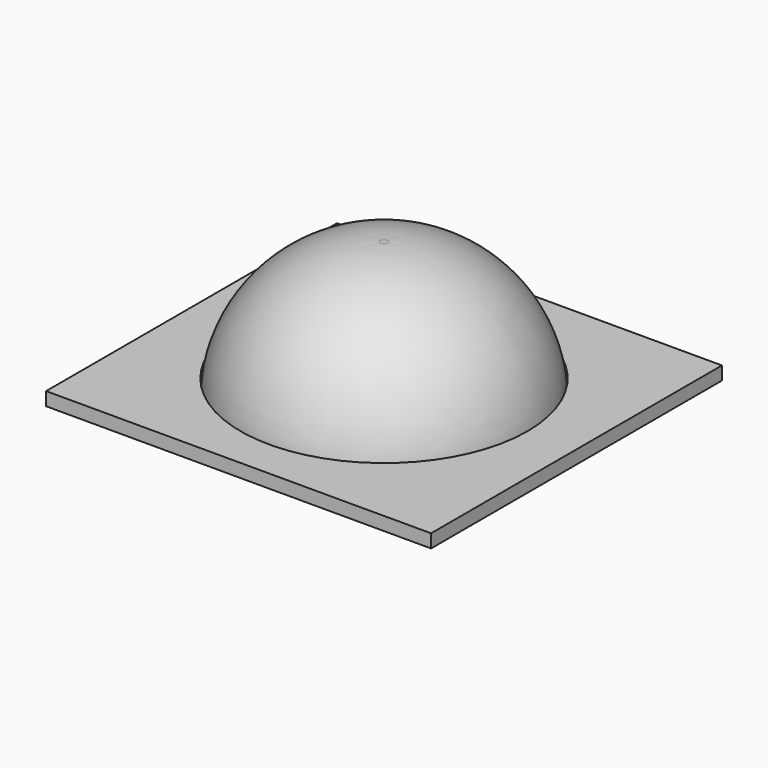
from build123d import *

# Parameters (mm, degrees)
F0_R     = 10.7488151117
F1_DEPTH = 10
F1_TAPER = -3
F3_W     = 28.8420915604
F3_H     = 27.2397696972
F3_R     = 10.7488151117
F4_DEPTH = 1


# Not quite as in the source:
# - a fillet or chamfer that OpenCascade refuses, or shapes differently, is made with other operations: its cross-section is extruded or revolved along the edge and cut away or added


with BuildPart() as f1:
    # F0 (on Top) → F1 (new body)
    with BuildSketch(Plane.XY):
        Circle(F0_R)
    extrude(amount=F1_DEPTH, taper=F1_TAPER)

    # F2: fillet of radius 10.5 on 1 edges, made by hand

    # F2_s1 → F2_t2 (revolve, cut)
    with BuildSketch(Plane.XZ):
        with BuildLine():
            ThreePointArc((10.7488151117, 0), (7.5064150031, 7.0993420768), (0.26072663, 10))
            Line((0.26072663, 10), (11.2728929045, 10))
            Line((11.2728929045, 10), (10.7488151117, 0))
        make_face()
    revolve(axis=Axis((0, 0, 10), (0, 0, -1)), mode=Mode.SUBTRACT)


with BuildPart() as f4:
    # F3 (on face) → F4 (new body)
    with BuildSketch(Plane.XY):
        Rectangle(F3_W, F3_H)
        Circle(F3_R, mode=Mode.SUBTRACT)
    extrude(amount=F4_DEPTH)


solid = Compound([f1.part, f4.part])
